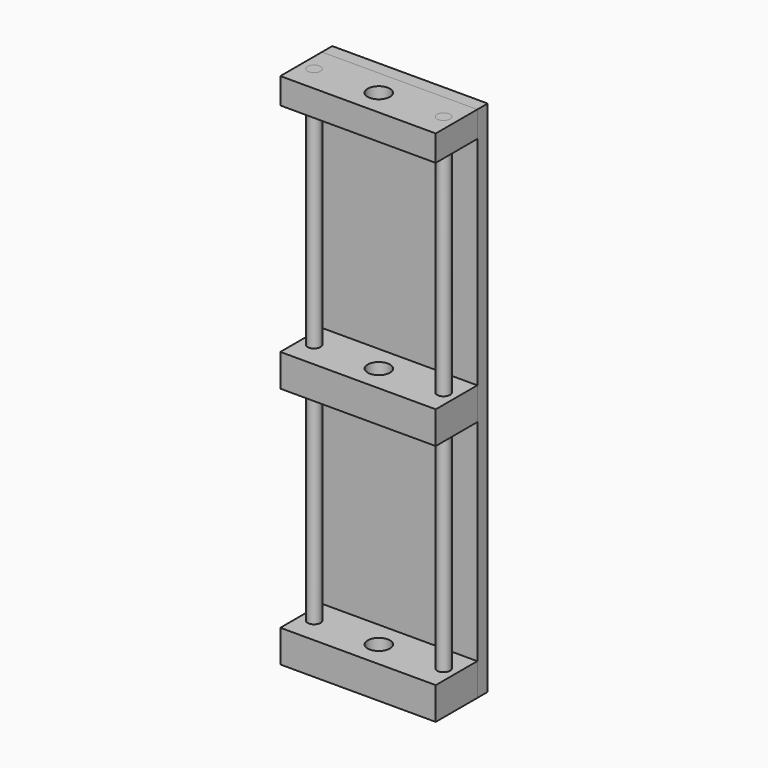
from build123d import *

# Parameters (mm, degrees)
F0_R     = 5
F1_DEPTH = 200
F2_W     = 120
F2_H     = 40.1148218211
F2_R     = 5
F2_R_2   = 8.6022132759
F4_DEPTH = 20
F3_W     = 120
F3_H     = 40.1148218211
F3_R     = 5
F3_R_2   = 8.6022132759
F5_DEPTH = 25
F6_W     = 120
F6_H     = 25
F7_DEPTH = 10
F6_H_2   = 20
F8_DEPTH = 355
F0_W     = 120
F0_H     = 40.1148218211
F0_R_2   = 8.6022132759
F9_DEPTH = 12.5


with BuildPart() as f1:
    # F0 (on Top) → F1 (new body, symmetric)
    with BuildSketch(Plane.XY):
        with Locations((-50, 0)):
            Circle(F0_R)
    extrude(amount=F1_DEPTH, both=True)


with BuildPart() as f1b:
    # F0 (on Top) → F1, piece 2 (new body, symmetric)
    with BuildSketch(Plane.XY):
        with BuildLine():
            ThreePointArc((45, 0), (50, -5), (55, 0))
            ThreePointArc((55, 0), (50, 5), (45, 0))
        make_face()
    extrude(amount=F1_DEPTH, both=True)


with BuildPart() as f4:
    # F2 (on face) → F4 (new body)
    with BuildSketch(Plane.XY.offset(200)):
        Rectangle(F2_W, F2_H)
        with Locations((-50, 0)):
            Circle(F2_R, mode=Mode.SUBTRACT)
        Circle(F2_R_2, mode=Mode.SUBTRACT)
        with Locations((50, 0)):
            Circle(F2_R, mode=Mode.SUBTRACT)
    extrude(amount=-F4_DEPTH)


with BuildPart() as f5:
    # F3 (on face) → F5 (new body)
    with BuildSketch(Plane(origin=(0, 0, -200), x_dir=(1, 0, 0), z_dir=(0, 0, -1))):
        Rectangle(F3_W, F3_H)
        with Locations((-50, 0)):
            Circle(F3_R, mode=Mode.SUBTRACT)
        Circle(F3_R_2, mode=Mode.SUBTRACT)
        with Locations((50, 0)):
            Circle(F3_R, mode=Mode.SUBTRACT)
    extrude(amount=-F5_DEPTH)


with BuildPart() as f7:
    # F6 (on face) → F7 (new body)
    with BuildSketch(Plane(origin=(0, 20.0574109105, 0), x_dir=(-1, 0, 0), z_dir=(0, 1, 0))):
        with Locations((0, -187.5)):
            Rectangle(F6_W, F6_H)
    extrude(amount=F7_DEPTH)

    # F8 (add, through all): a face of the model
    f8_faces = [f7.faces().sort_by_distance(p)[0] for p in [
        (0, 25.0574109105, -175),
    ]]


with BuildPart() as f7b:
    # F6 (on face) → F7, piece 2 (new body)
    with BuildSketch(Plane(origin=(0, 20.0574109105, 0), x_dir=(-1, 0, 0), z_dir=(0, 1, 0))):
        with Locations((0, 190)):
            Rectangle(F6_W, F6_H_2)
    extrude(amount=F7_DEPTH)


with BuildPart() as f7_1:
    add(f7.part)

    add(f7b.part)  # F8 merges F7b
    extrude(f8_faces, amount=F8_DEPTH)


with BuildPart() as f9:
    # F0 (on Top) → F9 (new body, symmetric)
    with BuildSketch(Plane.XY):
        Rectangle(F0_W, F0_H)
        with Locations((-50, 0)):
            Circle(F0_R, mode=Mode.SUBTRACT)
        Circle(F0_R_2, mode=Mode.SUBTRACT)
        with BuildLine():
            ThreePointArc((45, 0), (50, 5), (55, 0))
            ThreePointArc((55, 0), (50, -5), (45, 0))
        make_face(mode=Mode.SUBTRACT)
    extrude(amount=F9_DEPTH, both=True)


solid = Compound([f1.part, f1b.part, f4.part, f5.part, f7_1.part, f9.part])
